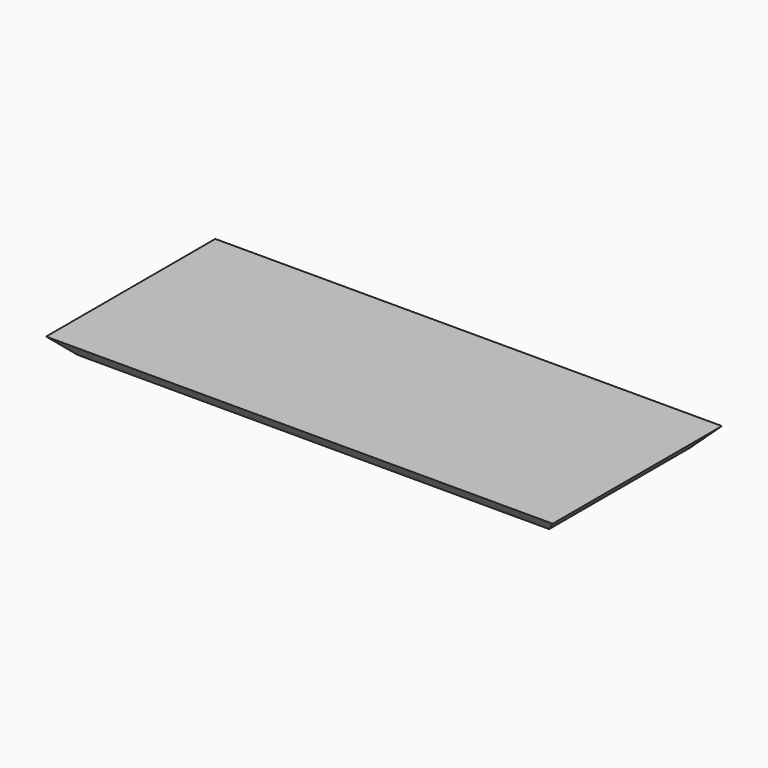
from build123d import *

# Parameters (mm, degrees)
F0_W     = 630
F0_H     = 263
F1_DEPTH = 22
F2_SIZE  = 21.99999


# Not quite as in the source:
# - a fillet or chamfer is up to 0.001 mm smaller than in the source, because OpenCascade refuses the exact size


with BuildPart() as f1:
    # F0 (on Top) → F1 (new body)
    with BuildSketch(Plane.XY):
        Rectangle(F0_W, F0_H)
    extrude(amount=F1_DEPTH)

    # F2 (size 22 in the source; OpenCascade refuses exactly that, so slightly less here)
    f2_edges = [f1.edges().sort_by_distance(p)[0] for p in [
        (0, 131.5, 0),
        (315, 0, 0),
        (0, -131.5, 0),
        (-315, 0, 0),
    ]]
    chamfer(f2_edges, length=F2_SIZE)


solid = f1.part
